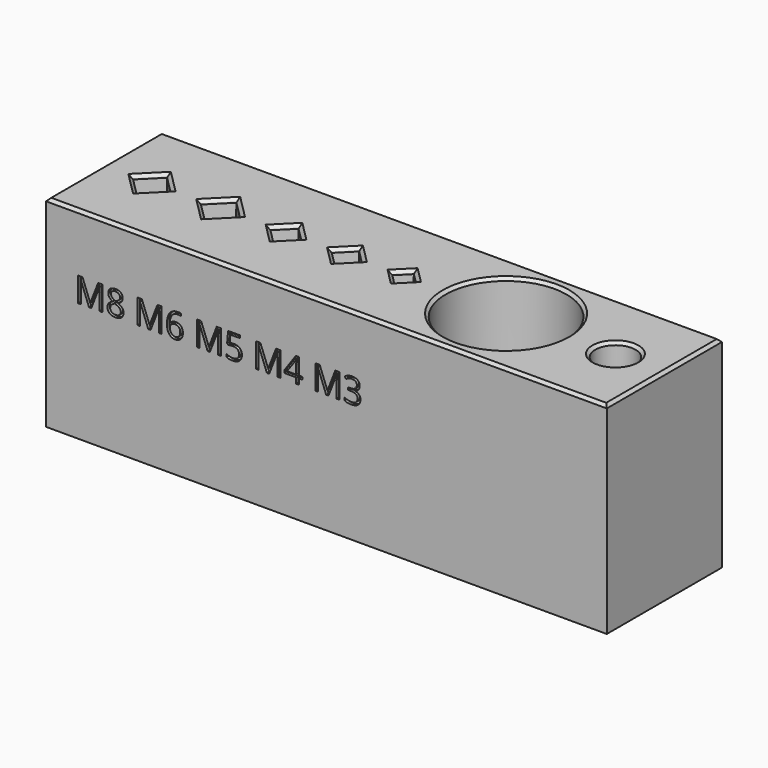
from build123d import *

# Parameters (mm, degrees)
F0_W          = 97.4156420974
F0_H          = 25
F0_R          = 10.5
F0_R_2        = 3.5
F1_DEPTH      = 13
F2_W          = 97.4156420974
F2_H          = 25
F2_R          = 10.5
F2_R_2        = 3.5
F3_DEPTH      = 20
F4_SIZE       = 0.5
F5_W          = 97.4156420974
F5_H          = 25
F6_DEPTH      = 2
F7_SIZE       = 3
F8_T4_DEPTH   = 49.6859183731
F8_T9_DEPTH   = 5
F8_T14_DEPTH  = 49.6859183731
F8_T19_DEPTH  = 49.6859183731
F8_T24_DEPTH  = 5
F8_T29_DEPTH  = 49.6859183731
F8_T34_DEPTH  = 49.6859183731
F8_T39_DEPTH  = 5
F8_T44_DEPTH  = 49.6859183731
F8_T49_DEPTH  = 49.6859183731
F8_T54_DEPTH  = 5
F8_T59_DEPTH  = 49.6859183731
F8_T64_DEPTH  = 48.6859183731
F8_T69_DEPTH  = 4
F8_T74_DEPTH  = 48.6859183731
F8_T79_DEPTH  = 48.6859183731
F8_T84_DEPTH  = 4
F8_T89_DEPTH  = 48.6859183731
F8_T94_DEPTH  = 48.6859183731
F8_T99_DEPTH  = 4
F8_T104_DEPTH = 48.6859183731
F8_T109_DEPTH = 48.6859183731
F8_T114_DEPTH = 4
F8_T119_DEPTH = 48.6859183731
F8_T124_DEPTH = 48.5859183731
F8_T129_DEPTH = 3.9
F8_T134_DEPTH = 48.5859183731
F8_T139_DEPTH = 48.5859183731
F8_T144_DEPTH = 3.9
F8_T149_DEPTH = 48.5859183731
F8_T154_DEPTH = 48.5859183731
F8_T159_DEPTH = 3.9
F8_T164_DEPTH = 48.5859183731
F8_T169_DEPTH = 48.5859183731
F8_T174_DEPTH = 3.9
F8_T179_DEPTH = 48.5859183731
F8_T184_DEPTH = 47.7859183731
F8_T189_DEPTH = 3.1
F8_T194_DEPTH = 47.7859183731
F8_T199_DEPTH = 47.7859183731
F8_T204_DEPTH = 3.1
F8_T209_DEPTH = 47.7859183731
F8_T214_DEPTH = 47.7859183731
F8_T219_DEPTH = 3.1
F8_T224_DEPTH = 47.7859183731
F8_T229_DEPTH = 47.7859183731
F8_T234_DEPTH = 3.1
F8_T239_DEPTH = 47.7859183731
F8_T244_DEPTH = 4.8
F8_T249_DEPTH = 4.8
F8_T254_DEPTH = 49.4859183731
F8_T259_DEPTH = 49.4859183731
F8_T264_DEPTH = 4.8
F8_T269_DEPTH = 49.4859183731
F8_T274_DEPTH = 49.4859183731
F8_T279_DEPTH = 4.8
F8_T284_DEPTH = 49.4859183731
F8_T289_DEPTH = 49.4859183731
F8_T294_DEPTH = 4.8
F8_T299_DEPTH = 4.8
F9_TEXT_SIZE  = 5.9394546838
F10_DEPTH     = 0.5


# Not quite as in the source:
# - a fillet or chamfer that OpenCascade refuses, or shapes differently, is made with other operations: its cross-section is extruded or revolved along the edge and cut away or added
# - Text() gives the source's letters only with a copy of the font that has no kerning and outlines rounded to 1/6400 em; it was checked with that copy


with BuildPart() as f1:
    # F0 (on Top) → F1 (new body)
    with BuildSketch(Plane.XY):
        with Locations((38.0792391653, 0)):
            Rectangle(F0_W, F0_H)
        Polygon((18.2307110279, 0), (21.0591381526, 2.8284271247), (23.8875652774, 0), (21.0591381526, -2.8284271247), align=None, mode=Mode.SUBTRACT)
        Polygon((-5.6285818834, 0), (-2.2344693337, 3.3941125497), (1.159643216, 0), (-2.2344693337, -3.3941125497), align=None, mode=Mode.SUBTRACT)
        Polygon((6.159643216, 0), (9.6951771219, 3.5355339059), (13.2307110279, 0), (9.6951771219, -3.5355339059), align=None, mode=Mode.SUBTRACT)
        Polygon((28.8875652774, 0), (31.645281724, 2.7577164466), (34.4029981706, 0), (31.645281724, -2.7577164466), align=None, mode=Mode.SUBTRACT)
        Polygon((39.4029981706, 0), (41.5950291923, 2.1920310217), (43.787060214, 0), (41.5950291923, -2.1920310217), align=None, mode=Mode.SUBTRACT)
        with Locations((59.287060214, 0)):
            Circle(F0_R, mode=Mode.SUBTRACT)
        with Locations((78.287060214, 0)):
            Circle(F0_R_2, mode=Mode.SUBTRACT)
    extrude(amount=F1_DEPTH)

    # F2 (on face) → F3 (join)
    with BuildSketch(Plane(origin=(0, 0, 0), x_dir=(1, 0, 0), z_dir=(0, 0, -1))):
        with Locations((38.0792391653, 0)):
            Rectangle(F2_W, F2_H)
        Polygon((1.159643216, 0), (-2.2344693337, -3.3941125497), (-5.6285818834, 0), (-2.2344693337, 3.3941125497), align=None, mode=Mode.SUBTRACT)
        Polygon((6.159643216, 0), (9.6951771219, 3.5355339059), (13.2307110279, 0), (9.6951771219, -3.5355339059), align=None, mode=Mode.SUBTRACT)
        Polygon((34.4029981706, 0), (31.645281724, -2.7577164466), (28.8875652774, 0), (31.645281724, 2.7577164466), align=None, mode=Mode.SUBTRACT)
        Polygon((41.5950291923, 2.1920310217), (43.787060214, 0), (41.5950291923, -2.1920310217), (39.4029981706, 0), align=None, mode=Mode.SUBTRACT)
        Polygon((23.8875652774, 0), (21.0591381526, -2.8284271247), (18.2307110279, 0), (21.0591381526, 2.8284271247), align=None, mode=Mode.SUBTRACT)
        with Locations((59.287060214, 0)):
            Circle(F2_R, mode=Mode.SUBTRACT)
        with Locations((78.287060214, 0)):
            Circle(F2_R_2, mode=Mode.SUBTRACT)
        Polygon((13.2307110279, 0), (9.6951771219, 3.5355339059), (6.159643216, 0), (9.6951771219, -3.5355339059), align=None)
        Polygon((-5.6285818834, 0), (-2.2344693337, -3.3941125497), (1.159643216, 0), (-2.2344693337, 3.3941125497), align=None)
        Polygon((18.2307110279, 0), (21.0591381526, -2.8284271247), (23.8875652774, 0), (21.0591381526, 2.8284271247), align=None)
        Polygon((28.8875652774, 0), (31.645281724, -2.7577164466), (34.4029981706, 0), (31.645281724, 2.7577164466), align=None)
        Polygon((41.5950291923, -2.1920310217), (43.787060214, 0), (41.5950291923, 2.1920310217), (39.4029981706, 0), align=None)
    extrude(amount=F3_DEPTH)

    # F4
    f4_edges = [f1.edges().sort_by_distance(p)[0] for p in [
        (38.079239, -12.5, 13),
        (86.78706, 0, 13),
        (38.079239, 12.5, 13),
        (-10.628582, 0, 13),
        (19.644925, 1.414214, 13),
        (22.473352, 1.414214, 13),
        (22.473352, -1.414214, 13),
        (19.644925, -1.414214, 13),
        (-3.931526, 1.697056, 13),
        (-0.537413, 1.697056, 13),
        (-0.537413, -1.697056, 13),
        (-3.931526, -1.697056, 13),
        (11.462944, -1.767767, 13),
        (7.92741, -1.767767, 13),
        (7.92741, 1.767767, 13),
        (11.462944, 1.767767, 13),
        (30.266424, 1.378858, 13),
        (33.02414, 1.378858, 13),
        (33.02414, -1.378858, 13),
        (30.266424, -1.378858, 13),
        (42.691045, 1.096016, 13),
        (42.691045, -1.096016, 13),
        (40.499014, -1.096016, 13),
        (40.499014, 1.096016, 13),
        (48.78706, 0, 13),
        (74.78706, 0, 13),
    ]]
    chamfer(f4_edges, length=F4_SIZE)

    # F5 (on face) → F6 (join)
    with BuildSketch(Plane(origin=(0, 0, -20), x_dir=(1, 0, 0), z_dir=(0, 0, -1))):
        with Locations((38.0792391653, 0)):
            Rectangle(F5_W, F5_H)
    extrude(amount=F6_DEPTH)

    # F7
    f7_edges = [f1.edges().sort_by_distance(p)[0] for p in [
        (48.78706, 0, -20),
    ]]
    chamfer(f7_edges, length=F7_SIZE)

    # F8: chamfer of 0.3 x 17.1869884892 on 21 edges, made by hand


with BuildPart() as f8_tool2:
    # F8_s3 → F8_t4 (new body)
    with BuildSketch(Plane(origin=(3.079821608, -3.079821608, 0), x_dir=(0, 0, 1), z_dir=(0.7071067812, -0.7071067812, 0))):
        Polygon((17.1869884892, -9.3555254877), (0, -9.0555254877), (0, -9.3555254877), align=None)
    extrude(amount=F8_T4_DEPTH)

    split(bisect_by=Plane(origin=(5.9593281864, -5.9593281864, 8.4277627439), x_dir=(-0.7071067812, -0.7071067812, 0), z_dir=(-0.5, 0.5, -0.7071067812)), keep=Keep.TOP)


with BuildPart() as f1_1:
    add(f1.part)

    # F8_t1: union F8_tool2
    add(f8_tool2.part)


with BuildPart() as f8_tool7:
    # F8_s8 → F8_t9 (new body)
    with BuildSketch(Plane(origin=(3.079821608, -3.079821608, 0), x_dir=(0, 0, 1), z_dir=(0.7071067812, -0.7071067812, 0))):
        Polygon((17.1869884892, -9.3555254877), (0, -9.0555254877), (0, -9.3555254877), align=None)
    extrude(amount=F8_T9_DEPTH)

    split(bisect_by=Plane(origin=(-1.1117396254, -1.1117396254, 1.5722372561), x_dir=(-0.7071067812, 0.7071067812, 0), z_dir=(0.5, 0.5, -0.7071067812)), keep=Keep.TOP)


with BuildPart() as f1_2:
    add(f1_1.part)

    # F8_t6: union F8_tool7
    add(f8_tool7.part)


with BuildPart() as f8_tool12:
    # F8_s13 → F8_t14 (new body)
    with BuildSketch(Plane(origin=(-28.5178942971, 28.5178942971, 0), x_dir=(0, 0, 1), z_dir=(0.7071067812, -0.7071067812, 0))):
        Polygon((17.1869884892, -9.3555254877), (0, -9.0555254877), (0, -9.3555254877), align=None)
    extrude(amount=F8_T14_DEPTH)

    split(bisect_by=Plane(origin=(-1.1117396254, 1.1117396254, 1.5722372561), x_dir=(0.7071067812, 0.7071067812, 0), z_dir=(0.5, -0.5, -0.7071067812)), keep=Keep.TOP)


with BuildPart() as f1_3:
    add(f1_2.part)

    # F8_t11: union F8_tool12
    add(f8_tool12.part)


with BuildPart() as f8_tool17:
    # F8_s18 → F8_t19 (new body)
    with BuildSketch(Plane(origin=(3.079821608, 3.079821608, 0), x_dir=(0, 0, 1), z_dir=(0.7071067812, 0.7071067812, 0))):
        Polygon((17.1869884892, 4.3555254877), (0, 4.6555254877), (0, 4.3555254877), align=None)
    extrude(amount=F8_T19_DEPTH)

    split(bisect_by=Plane(origin=(5.9593281864, 5.9593281864, 8.4277627439), x_dir=(0.7071067812, -0.7071067812, 0), z_dir=(-0.5, -0.5, -0.7071067812)), keep=Keep.TOP)


with BuildPart() as f1_4:
    add(f1_3.part)

    # F8_t16: union F8_tool17
    add(f8_tool17.part)


with BuildPart() as f8_tool22:
    # F8_s23 → F8_t24 (new body)
    with BuildSketch(Plane(origin=(3.079821608, 3.079821608, 0), x_dir=(0, 0, 1), z_dir=(0.7071067812, 0.7071067812, 0))):
        Polygon((17.1869884892, 4.3555254877), (0, 4.6555254877), (0, 4.3555254877), align=None)
    extrude(amount=F8_T24_DEPTH)

    split(bisect_by=Plane(origin=(5.9593281864, -5.9593281864, 8.4277627439), x_dir=(-0.7071067812, -0.7071067812, 0), z_dir=(-0.5, 0.5, -0.7071067812)), keep=Keep.TOP)


with BuildPart() as f1_5:
    add(f1_4.part)

    # F8_t21: union F8_tool22
    add(f8_tool22.part)


with BuildPart() as f8_tool27:
    # F8_s28 → F8_t29 (new body)
    with BuildSketch(Plane(origin=(-28.5178942971, -28.5178942971, 0), x_dir=(0, 0, 1), z_dir=(0.7071067812, 0.7071067812, 0))):
        Polygon((17.1869884892, 4.3555254877), (0, 4.6555254877), (0, 4.3555254877), align=None)
    extrude(amount=F8_T29_DEPTH)

    split(bisect_by=Plane(origin=(-1.1117396254, -1.1117396254, 1.5722372561), x_dir=(-0.7071067812, 0.7071067812, 0), z_dir=(0.5, 0.5, -0.7071067812)), keep=Keep.TOP)


with BuildPart() as f1_6:
    add(f1_5.part)

    # F8_t26: union F8_tool27
    add(f8_tool27.part)


with BuildPart() as f8_tool32:
    # F8_s33 → F8_t34 (new body)
    with BuildSketch(Plane(origin=(6.6153555139, -6.6153555139, 0), x_dir=(0, 0, 1), z_dir=(-0.7071067812, 0.7071067812, 0))):
        Polygon((17.1869884892, 4.3555254877), (0, 4.6555254877), (0, 4.3555254877), align=None)
    extrude(amount=F8_T34_DEPTH)

    split(bisect_by=Plane(origin=(-1.1117396254, 1.1117396254, 1.5722372561), x_dir=(0.7071067812, 0.7071067812, 0), z_dir=(0.5, -0.5, -0.7071067812)), keep=Keep.TOP)


with BuildPart() as f1_7:
    add(f1_6.part)

    # F8_t31: union F8_tool32
    add(f8_tool32.part)


with BuildPart() as f8_tool37:
    # F8_s38 → F8_t39 (new body)
    with BuildSketch(Plane(origin=(6.6153555139, -6.6153555139, 0), x_dir=(0, 0, 1), z_dir=(-0.7071067812, 0.7071067812, 0))):
        Polygon((17.1869884892, 4.3555254877), (0, 4.6555254877), (0, 4.3555254877), align=None)
    extrude(amount=F8_T39_DEPTH)

    split(bisect_by=Plane(origin=(5.9593281864, 5.9593281864, 8.4277627439), x_dir=(0.7071067812, -0.7071067812, 0), z_dir=(-0.5, -0.5, -0.7071067812)), keep=Keep.TOP)


with BuildPart() as f1_8:
    add(f1_7.part)

    # F8_t36: union F8_tool37
    add(f8_tool37.part)


with BuildPart() as f8_tool42:
    # F8_s43 → F8_t44 (new body)
    with BuildSketch(Plane(origin=(38.2130714191, -38.2130714191, 0), x_dir=(0, 0, 1), z_dir=(-0.7071067812, 0.7071067812, 0))):
        Polygon((17.1869884892, 4.3555254877), (0, 4.6555254877), (0, 4.3555254877), align=None)
    extrude(amount=F8_T44_DEPTH)

    split(bisect_by=Plane(origin=(5.9593281864, -5.9593281864, 8.4277627439), x_dir=(-0.7071067812, -0.7071067812, 0), z_dir=(-0.5, 0.5, -0.7071067812)), keep=Keep.TOP)


with BuildPart() as f1_9:
    add(f1_8.part)

    # F8_t41: union F8_tool42
    add(f8_tool42.part)


with BuildPart() as f8_tool47:
    # F8_s48 → F8_t49 (new body)
    with BuildSketch(Plane(origin=(6.6153555139, 6.6153555139, 0), x_dir=(0, 0, 1), z_dir=(-0.7071067812, -0.7071067812, 0))):
        Polygon((17.1869884892, -9.3555254877), (0, -9.0555254877), (0, -9.3555254877), align=None)
    extrude(amount=F8_T49_DEPTH)

    split(bisect_by=Plane(origin=(-1.1117396254, -1.1117396254, 1.5722372561), x_dir=(-0.7071067812, 0.7071067812, 0), z_dir=(0.5, 0.5, -0.7071067812)), keep=Keep.TOP)


with BuildPart() as f1_10:
    add(f1_9.part)

    # F8_t46: union F8_tool47
    add(f8_tool47.part)


with BuildPart() as f8_tool52:
    # F8_s53 → F8_t54 (new body)
    with BuildSketch(Plane(origin=(6.6153555139, 6.6153555139, 0), x_dir=(0, 0, 1), z_dir=(-0.7071067812, -0.7071067812, 0))):
        Polygon((17.1869884892, -9.3555254877), (0, -9.0555254877), (0, -9.3555254877), align=None)
    extrude(amount=F8_T54_DEPTH)

    split(bisect_by=Plane(origin=(-1.1117396254, 1.1117396254, 1.5722372561), x_dir=(0.7071067812, 0.7071067812, 0), z_dir=(0.5, -0.5, -0.7071067812)), keep=Keep.TOP)


with BuildPart() as f1_11:
    add(f1_10.part)

    # F8_t51: union F8_tool52
    add(f8_tool52.part)


with BuildPart() as f8_tool57:
    # F8_s58 → F8_t59 (new body)
    with BuildSketch(Plane(origin=(38.2130714191, 38.2130714191, 0), x_dir=(0, 0, 1), z_dir=(-0.7071067812, -0.7071067812, 0))):
        Polygon((17.1869884892, -9.3555254877), (0, -9.0555254877), (0, -9.3555254877), align=None)
    extrude(amount=F8_T59_DEPTH)

    split(bisect_by=Plane(origin=(5.9593281864, 5.9593281864, 8.4277627439), x_dir=(0.7071067812, -0.7071067812, 0), z_dir=(-0.5, -0.5, -0.7071067812)), keep=Keep.TOP)


with BuildPart() as f1_12:
    add(f1_11.part)

    # F8_t56: union F8_tool57
    add(f8_tool57.part)


with BuildPart() as f8_tool62:
    # F8_s63 → F8_t64 (new body)
    with BuildSketch(Plane(origin=(11.9437826387, -11.9437826387, 0), x_dir=(0, 0, 1), z_dir=(-0.7071067812, 0.7071067812, 0))):
        Polygon((17.1869884892, 12.8910593937), (0, 13.1910593937), (0, 12.8910593937), align=None)
    extrude(amount=F8_T64_DEPTH)

    split(bisect_by=Plane(origin=(1.5524739369, -1.5524739369, -2.1955296968), x_dir=(0.7071067812, 0.7071067812, 0), z_dir=(0.5, -0.5, -0.7071067812)), keep=Keep.TOP)


with BuildPart() as f1_13:
    add(f1_12.part)

    # F8_t61: union F8_tool62
    add(f8_tool62.part)


with BuildPart() as f8_tool67:
    # F8_s68 → F8_t69 (new body)
    with BuildSketch(Plane(origin=(11.9437826387, -11.9437826387, 0), x_dir=(0, 0, 1), z_dir=(-0.7071067812, 0.7071067812, 0))):
        Polygon((17.1869884892, 12.8910593937), (0, 13.1910593937), (0, 12.8910593937), align=None)
    extrude(amount=F8_T69_DEPTH)

    split(bisect_by=Plane(origin=(8.9770951394, 8.9770951394, 12.6955296968), x_dir=(0.7071067812, -0.7071067812, 0), z_dir=(-0.5, -0.5, -0.7071067812)), keep=Keep.TOP)


with BuildPart() as f1_14:
    add(f1_13.part)

    # F8_t66: union F8_tool67
    add(f8_tool67.part)


with BuildPart() as f8_tool72:
    # F8_s73 → F8_t74 (new body)
    with BuildSketch(Plane(origin=(43.5414985438, -43.5414985438, 0), x_dir=(0, 0, 1), z_dir=(-0.7071067812, 0.7071067812, 0))):
        Polygon((17.1869884892, 12.8910593937), (0, 13.1910593937), (0, 12.8910593937), align=None)
    extrude(amount=F8_T74_DEPTH)

    split(bisect_by=Plane(origin=(8.9770951394, -8.9770951394, 12.6955296968), x_dir=(-0.7071067812, -0.7071067812, 0), z_dir=(-0.5, 0.5, -0.7071067812)), keep=Keep.TOP)


with BuildPart() as f1_15:
    add(f1_14.part)

    # F8_t71: union F8_tool72
    add(f8_tool72.part)


with BuildPart() as f8_tool77:
    # F8_s78 → F8_t79 (new body)
    with BuildSketch(Plane(origin=(11.9437826387, 11.9437826387, 0), x_dir=(0, 0, 1), z_dir=(-0.7071067812, -0.7071067812, 0))):
        Polygon((17.1869884892, -16.8910593937), (0, -16.5910593937), (0, -16.8910593937), align=None)
    extrude(amount=F8_T79_DEPTH)

    split(bisect_by=Plane(origin=(1.5524739369, 1.5524739369, -2.1955296968), x_dir=(-0.7071067812, 0.7071067812, 0), z_dir=(0.5, 0.5, -0.7071067812)), keep=Keep.TOP)


with BuildPart() as f1_16:
    add(f1_15.part)

    # F8_t76: union F8_tool77
    add(f8_tool77.part)


with BuildPart() as f8_tool82:
    # F8_s83 → F8_t84 (new body)
    with BuildSketch(Plane(origin=(11.9437826387, 11.9437826387, 0), x_dir=(0, 0, 1), z_dir=(-0.7071067812, -0.7071067812, 0))):
        Polygon((17.1869884892, -16.8910593937), (0, -16.5910593937), (0, -16.8910593937), align=None)
    extrude(amount=F8_T84_DEPTH)

    split(bisect_by=Plane(origin=(1.5524739369, -1.5524739369, -2.1955296968), x_dir=(0.7071067812, 0.7071067812, 0), z_dir=(0.5, -0.5, -0.7071067812)), keep=Keep.TOP)


with BuildPart() as f1_17:
    add(f1_16.part)

    # F8_t81: union F8_tool82
    add(f8_tool82.part)


with BuildPart() as f8_tool87:
    # F8_s88 → F8_t89 (new body)
    with BuildSketch(Plane(origin=(43.5414985438, 43.5414985438, 0), x_dir=(0, 0, 1), z_dir=(-0.7071067812, -0.7071067812, 0))):
        Polygon((17.1869884892, -16.8910593937), (0, -16.5910593937), (0, -16.8910593937), align=None)
    extrude(amount=F8_T89_DEPTH)

    split(bisect_by=Plane(origin=(8.9770951394, 8.9770951394, 12.6955296968), x_dir=(0.7071067812, -0.7071067812, 0), z_dir=(-0.5, -0.5, -0.7071067812)), keep=Keep.TOP)


with BuildPart() as f1_18:
    add(f1_17.part)

    # F8_t86: union F8_tool87
    add(f8_tool87.part)


with BuildPart() as f8_tool92:
    # F8_s93 → F8_t94 (new body)
    with BuildSketch(Plane(origin=(9.1153555139, -9.1153555139, 0), x_dir=(0, 0, 1), z_dir=(0.7071067812, -0.7071067812, 0))):
        Polygon((17.1869884892, -16.8910593937), (0, -16.5910593937), (0, -16.8910593937), align=None)
    extrude(amount=F8_T94_DEPTH)

    split(bisect_by=Plane(origin=(8.9770951394, -8.9770951394, 12.6955296968), x_dir=(-0.7071067812, -0.7071067812, 0), z_dir=(-0.5, 0.5, -0.7071067812)), keep=Keep.TOP)


with BuildPart() as f1_19:
    add(f1_18.part)

    # F8_t91: union F8_tool92
    add(f8_tool92.part)


with BuildPart() as f8_tool97:
    # F8_s98 → F8_t99 (new body)
    with BuildSketch(Plane(origin=(9.1153555139, -9.1153555139, 0), x_dir=(0, 0, 1), z_dir=(0.7071067812, -0.7071067812, 0))):
        Polygon((17.1869884892, -16.8910593937), (0, -16.5910593937), (0, -16.8910593937), align=None)
    extrude(amount=F8_T99_DEPTH)

    split(bisect_by=Plane(origin=(1.5524739369, 1.5524739369, -2.1955296968), x_dir=(-0.7071067812, 0.7071067812, 0), z_dir=(0.5, 0.5, -0.7071067812)), keep=Keep.TOP)


with BuildPart() as f1_20:
    add(f1_19.part)

    # F8_t96: union F8_tool97
    add(f8_tool97.part)


with BuildPart() as f8_tool102:
    # F8_s103 → F8_t104 (new body)
    with BuildSketch(Plane(origin=(-22.4823603912, 22.4823603912, 0), x_dir=(0, 0, 1), z_dir=(0.7071067812, -0.7071067812, 0))):
        Polygon((17.1869884892, -16.8910593937), (0, -16.5910593937), (0, -16.8910593937), align=None)
    extrude(amount=F8_T104_DEPTH)

    split(bisect_by=Plane(origin=(1.5524739369, -1.5524739369, -2.1955296968), x_dir=(0.7071067812, 0.7071067812, 0), z_dir=(0.5, -0.5, -0.7071067812)), keep=Keep.TOP)


with BuildPart() as f1_21:
    add(f1_20.part)

    # F8_t101: union F8_tool102
    add(f8_tool102.part)


with BuildPart() as f8_tool107:
    # F8_s108 → F8_t109 (new body)
    with BuildSketch(Plane(origin=(9.1153555139, 9.1153555139, 0), x_dir=(0, 0, 1), z_dir=(0.7071067812, 0.7071067812, 0))):
        Polygon((17.1869884892, 12.8910593937), (0, 13.1910593937), (0, 12.8910593937), align=None)
    extrude(amount=F8_T109_DEPTH)

    split(bisect_by=Plane(origin=(8.9770951394, 8.9770951394, 12.6955296968), x_dir=(0.7071067812, -0.7071067812, 0), z_dir=(-0.5, -0.5, -0.7071067812)), keep=Keep.TOP)


with BuildPart() as f1_22:
    add(f1_21.part)

    # F8_t106: union F8_tool107
    add(f8_tool107.part)


with BuildPart() as f8_tool112:
    # F8_s113 → F8_t114 (new body)
    with BuildSketch(Plane(origin=(9.1153555139, 9.1153555139, 0), x_dir=(0, 0, 1), z_dir=(0.7071067812, 0.7071067812, 0))):
        Polygon((17.1869884892, 12.8910593937), (0, 13.1910593937), (0, 12.8910593937), align=None)
    extrude(amount=F8_T114_DEPTH)

    split(bisect_by=Plane(origin=(8.9770951394, -8.9770951394, 12.6955296968), x_dir=(-0.7071067812, -0.7071067812, 0), z_dir=(-0.5, 0.5, -0.7071067812)), keep=Keep.TOP)


with BuildPart() as f1_23:
    add(f1_22.part)

    # F8_t111: union F8_tool112
    add(f8_tool112.part)


with BuildPart() as f8_tool117:
    # F8_s118 → F8_t119 (new body)
    with BuildSketch(Plane(origin=(-22.4823603912, -22.4823603912, 0), x_dir=(0, 0, 1), z_dir=(0.7071067812, 0.7071067812, 0))):
        Polygon((17.1869884892, 12.8910593937), (0, 13.1910593937), (0, 12.8910593937), align=None)
    extrude(amount=F8_T119_DEPTH)

    split(bisect_by=Plane(origin=(1.5524739369, 1.5524739369, -2.1955296968), x_dir=(-0.7071067812, 0.7071067812, 0), z_dir=(0.5, 0.5, -0.7071067812)), keep=Keep.TOP)


with BuildPart() as f1_24:
    add(f1_23.part)

    # F8_t116: union F8_tool117
    add(f8_tool117.part)


with BuildPart() as f8_tool122:
    # F8_s123 → F8_t124 (new body)
    with BuildSketch(Plane(origin=(17.2014990853, -17.2014990853, 0), x_dir=(0, 0, 1), z_dir=(-0.7071067812, 0.7071067812, 0))):
        Polygon((17.1869884892, 20.4265932996), (0, 20.7265932996), (0, 20.4265932996), align=None)
    extrude(amount=F8_T124_DEPTH)

    split(bisect_by=Plane(origin=(4.1813321602, -4.1813321602, -5.9132966498), x_dir=(0.7071067812, 0.7071067812, 0), z_dir=(0.5, -0.5, -0.7071067812)), keep=Keep.TOP)


with BuildPart() as f1_25:
    add(f1_24.part)

    # F8_t121: union F8_tool122
    add(f8_tool122.part)


with BuildPart() as f8_tool127:
    # F8_s128 → F8_t129 (new body)
    with BuildSketch(Plane(origin=(17.2014990853, -17.2014990853, 0), x_dir=(0, 0, 1), z_dir=(-0.7071067812, 0.7071067812, 0))):
        Polygon((17.1869884892, 20.4265932996), (0, 20.7265932996), (0, 20.4265932996), align=None)
    extrude(amount=F8_T129_DEPTH)

    split(bisect_by=Plane(origin=(11.6413087018, 11.6413087018, 16.4632966498), x_dir=(0.7071067812, -0.7071067812, 0), z_dir=(-0.5, -0.5, -0.7071067812)), keep=Keep.TOP)


with BuildPart() as f1_26:
    add(f1_25.part)

    # F8_t126: union F8_tool127
    add(f8_tool127.part)


with BuildPart() as f8_tool132:
    # F8_s133 → F8_t134 (new body)
    with BuildSketch(Plane(origin=(48.7992149904, -48.7992149904, 0), x_dir=(0, 0, 1), z_dir=(-0.7071067812, 0.7071067812, 0))):
        Polygon((17.1869884892, 20.4265932996), (0, 20.7265932996), (0, 20.4265932996), align=None)
    extrude(amount=F8_T134_DEPTH)

    split(bisect_by=Plane(origin=(11.6413087018, -11.6413087018, 16.4632966498), x_dir=(-0.7071067812, -0.7071067812, 0), z_dir=(-0.5, 0.5, -0.7071067812)), keep=Keep.TOP)


with BuildPart() as f1_27:
    add(f1_26.part)

    # F8_t131: union F8_tool132
    add(f8_tool132.part)


with BuildPart() as f8_tool137:
    # F8_s138 → F8_t139 (new body)
    with BuildSketch(Plane(origin=(17.2014990853, 17.2014990853, 0), x_dir=(0, 0, 1), z_dir=(-0.7071067812, -0.7071067812, 0))):
        Polygon((17.1869884892, -24.3265932996), (0, -24.0265932996), (0, -24.3265932996), align=None)
    extrude(amount=F8_T139_DEPTH)

    split(bisect_by=Plane(origin=(4.1813321602, 4.1813321602, -5.9132966498), x_dir=(-0.7071067812, 0.7071067812, 0), z_dir=(0.5, 0.5, -0.7071067812)), keep=Keep.TOP)


with BuildPart() as f1_28:
    add(f1_27.part)

    # F8_t136: union F8_tool137
    add(f8_tool137.part)


with BuildPart() as f8_tool142:
    # F8_s143 → F8_t144 (new body)
    with BuildSketch(Plane(origin=(17.2014990853, 17.2014990853, 0), x_dir=(0, 0, 1), z_dir=(-0.7071067812, -0.7071067812, 0))):
        Polygon((17.1869884892, -24.3265932996), (0, -24.0265932996), (0, -24.3265932996), align=None)
    extrude(amount=F8_T144_DEPTH)

    split(bisect_by=Plane(origin=(4.1813321602, -4.1813321602, -5.9132966498), x_dir=(0.7071067812, 0.7071067812, 0), z_dir=(0.5, -0.5, -0.7071067812)), keep=Keep.TOP)


with BuildPart() as f1_29:
    add(f1_28.part)

    # F8_t141: union F8_tool142
    add(f8_tool142.part)


with BuildPart() as f8_tool147:
    # F8_s148 → F8_t149 (new body)
    with BuildSketch(Plane(origin=(48.7992149904, 48.7992149904, 0), x_dir=(0, 0, 1), z_dir=(-0.7071067812, -0.7071067812, 0))):
        Polygon((17.1869884892, -24.3265932996), (0, -24.0265932996), (0, -24.3265932996), align=None)
    extrude(amount=F8_T149_DEPTH)

    split(bisect_by=Plane(origin=(11.6413087018, 11.6413087018, 16.4632966498), x_dir=(0.7071067812, -0.7071067812, 0), z_dir=(-0.5, -0.5, -0.7071067812)), keep=Keep.TOP)


with BuildPart() as f1_30:
    add(f1_29.part)

    # F8_t146: union F8_tool147
    add(f8_tool147.part)


with BuildPart() as f8_tool152:
    # F8_s153 → F8_t154 (new body)
    with BuildSketch(Plane(origin=(14.4437826387, -14.4437826387, 0), x_dir=(0, 0, 1), z_dir=(0.7071067812, -0.7071067812, 0))):
        Polygon((17.1869884892, -24.3265932996), (0, -24.0265932996), (0, -24.3265932996), align=None)
    extrude(amount=F8_T154_DEPTH)

    split(bisect_by=Plane(origin=(11.6413087018, -11.6413087018, 16.4632966498), x_dir=(-0.7071067812, -0.7071067812, 0), z_dir=(-0.5, 0.5, -0.7071067812)), keep=Keep.TOP)


with BuildPart() as f1_31:
    add(f1_30.part)

    # F8_t151: union F8_tool152
    add(f8_tool152.part)


with BuildPart() as f8_tool157:
    # F8_s158 → F8_t159 (new body)
    with BuildSketch(Plane(origin=(14.4437826387, -14.4437826387, 0), x_dir=(0, 0, 1), z_dir=(0.7071067812, -0.7071067812, 0))):
        Polygon((17.1869884892, -24.3265932996), (0, -24.0265932996), (0, -24.3265932996), align=None)
    extrude(amount=F8_T159_DEPTH)

    split(bisect_by=Plane(origin=(4.1813321602, 4.1813321602, -5.9132966498), x_dir=(-0.7071067812, 0.7071067812, 0), z_dir=(0.5, 0.5, -0.7071067812)), keep=Keep.TOP)


with BuildPart() as f1_32:
    add(f1_31.part)

    # F8_t156: union F8_tool157
    add(f8_tool157.part)


with BuildPart() as f8_tool162:
    # F8_s163 → F8_t164 (new body)
    with BuildSketch(Plane(origin=(-17.1539332665, 17.1539332665, 0), x_dir=(0, 0, 1), z_dir=(0.7071067812, -0.7071067812, 0))):
        Polygon((17.1869884892, -24.3265932996), (0, -24.0265932996), (0, -24.3265932996), align=None)
    extrude(amount=F8_T164_DEPTH)

    split(bisect_by=Plane(origin=(4.1813321602, -4.1813321602, -5.9132966498), x_dir=(0.7071067812, 0.7071067812, 0), z_dir=(0.5, -0.5, -0.7071067812)), keep=Keep.TOP)


with BuildPart() as f1_33:
    add(f1_32.part)

    # F8_t161: union F8_tool162
    add(f8_tool162.part)


with BuildPart() as f8_tool167:
    # F8_s168 → F8_t169 (new body)
    with BuildSketch(Plane(origin=(14.4437826387, 14.4437826387, 0), x_dir=(0, 0, 1), z_dir=(0.7071067812, 0.7071067812, 0))):
        Polygon((17.1869884892, 20.4265932996), (0, 20.7265932996), (0, 20.4265932996), align=None)
    extrude(amount=F8_T169_DEPTH)

    split(bisect_by=Plane(origin=(11.6413087018, 11.6413087018, 16.4632966498), x_dir=(0.7071067812, -0.7071067812, 0), z_dir=(-0.5, -0.5, -0.7071067812)), keep=Keep.TOP)


with BuildPart() as f1_34:
    add(f1_33.part)

    # F8_t166: union F8_tool167
    add(f8_tool167.part)


with BuildPart() as f8_tool172:
    # F8_s173 → F8_t174 (new body)
    with BuildSketch(Plane(origin=(14.4437826387, 14.4437826387, 0), x_dir=(0, 0, 1), z_dir=(0.7071067812, 0.7071067812, 0))):
        Polygon((17.1869884892, 20.4265932996), (0, 20.7265932996), (0, 20.4265932996), align=None)
    extrude(amount=F8_T174_DEPTH)

    split(bisect_by=Plane(origin=(11.6413087018, -11.6413087018, 16.4632966498), x_dir=(-0.7071067812, -0.7071067812, 0), z_dir=(-0.5, 0.5, -0.7071067812)), keep=Keep.TOP)


with BuildPart() as f1_35:
    add(f1_34.part)

    # F8_t171: union F8_tool172
    add(f8_tool172.part)


with BuildPart() as f8_tool177:
    # F8_s178 → F8_t179 (new body)
    with BuildSketch(Plane(origin=(-17.1539332665, -17.1539332665, 0), x_dir=(0, 0, 1), z_dir=(0.7071067812, 0.7071067812, 0))):
        Polygon((17.1869884892, 20.4265932996), (0, 20.7265932996), (0, 20.4265932996), align=None)
    extrude(amount=F8_T179_DEPTH)

    split(bisect_by=Plane(origin=(4.1813321602, 4.1813321602, -5.9132966498), x_dir=(-0.7071067812, 0.7071067812, 0), z_dir=(0.5, 0.5, -0.7071067812)), keep=Keep.TOP)


with BuildPart() as f1_36:
    add(f1_35.part)

    # F8_t176: union F8_tool177
    add(f8_tool177.part)


with BuildPart() as f8_tool182:
    # F8_s183 → F8_t184 (new body)
    with BuildSketch(Plane(origin=(19.7014990853, 19.7014990853, 0), x_dir=(0, 0, 1), z_dir=(0.7071067812, 0.7071067812, 0))):
        Polygon((17.1869884892, 27.8621272055), (0, 28.1621272055), (0, 27.8621272055), align=None)
    extrude(amount=F8_T184_DEPTH)

    split(bisect_by=Plane(origin=(14.2701669251, 14.2701669251, 20.1810636028), x_dir=(0.7071067812, -0.7071067812, 0), z_dir=(-0.5, -0.5, -0.7071067812)), keep=Keep.TOP)


with BuildPart() as f1_37:
    add(f1_36.part)

    # F8_t181: union F8_tool182
    add(f8_tool182.part)


with BuildPart() as f8_tool187:
    # F8_s188 → F8_t189 (new body)
    with BuildSketch(Plane(origin=(19.7014990853, 19.7014990853, 0), x_dir=(0, 0, 1), z_dir=(0.7071067812, 0.7071067812, 0))):
        Polygon((17.1869884892, 27.8621272055), (0, 28.1621272055), (0, 27.8621272055), align=None)
    extrude(amount=F8_T189_DEPTH)

    split(bisect_by=Plane(origin=(14.2701669251, -14.2701669251, 20.1810636028), x_dir=(-0.7071067812, -0.7071067812, 0), z_dir=(-0.5, 0.5, -0.7071067812)), keep=Keep.TOP)


with BuildPart() as f1_38:
    add(f1_37.part)

    # F8_t186: union F8_tool187
    add(f8_tool187.part)


with BuildPart() as f8_tool192:
    # F8_s193 → F8_t194 (new body)
    with BuildSketch(Plane(origin=(-11.8962168198, -11.8962168198, 0), x_dir=(0, 0, 1), z_dir=(0.7071067812, 0.7071067812, 0))):
        Polygon((17.1869884892, 27.8621272055), (0, 28.1621272055), (0, 27.8621272055), align=None)
    extrude(amount=F8_T194_DEPTH)

    split(bisect_by=Plane(origin=(6.5273476711, 6.5273476711, -9.2310636028), x_dir=(-0.7071067812, 0.7071067812, 0), z_dir=(0.5, 0.5, -0.7071067812)), keep=Keep.TOP)


with BuildPart() as f1_39:
    add(f1_38.part)

    # F8_t191: union F8_tool192
    add(f8_tool192.part)


with BuildPart() as f8_tool197:
    # F8_s198 → F8_t199 (new body)
    with BuildSketch(Plane(origin=(21.893530107, -21.893530107, 0), x_dir=(0, 0, 1), z_dir=(-0.7071067812, 0.7071067812, 0))):
        Polygon((17.1869884892, 27.8621272055), (0, 28.1621272055), (0, 27.8621272055), align=None)
    extrude(amount=F8_T199_DEPTH)

    split(bisect_by=Plane(origin=(6.5273476711, -6.5273476711, -9.2310636028), x_dir=(0.7071067812, 0.7071067812, 0), z_dir=(0.5, -0.5, -0.7071067812)), keep=Keep.TOP)


with BuildPart() as f1_40:
    add(f1_39.part)

    # F8_t196: union F8_tool197
    add(f8_tool197.part)


with BuildPart() as f8_tool202:
    # F8_s203 → F8_t204 (new body)
    with BuildSketch(Plane(origin=(21.893530107, -21.893530107, 0), x_dir=(0, 0, 1), z_dir=(-0.7071067812, 0.7071067812, 0))):
        Polygon((17.1869884892, 27.8621272055), (0, 28.1621272055), (0, 27.8621272055), align=None)
    extrude(amount=F8_T204_DEPTH)

    split(bisect_by=Plane(origin=(14.2701669251, 14.2701669251, 20.1810636028), x_dir=(0.7071067812, -0.7071067812, 0), z_dir=(-0.5, -0.5, -0.7071067812)), keep=Keep.TOP)


with BuildPart() as f1_41:
    add(f1_40.part)

    # F8_t201: union F8_tool202
    add(f8_tool202.part)


with BuildPart() as f8_tool207:
    # F8_s208 → F8_t209 (new body)
    with BuildSketch(Plane(origin=(53.4912460121, -53.4912460121, 0), x_dir=(0, 0, 1), z_dir=(-0.7071067812, 0.7071067812, 0))):
        Polygon((17.1869884892, 27.8621272055), (0, 28.1621272055), (0, 27.8621272055), align=None)
    extrude(amount=F8_T209_DEPTH)

    split(bisect_by=Plane(origin=(14.2701669251, -14.2701669251, 20.1810636028), x_dir=(-0.7071067812, -0.7071067812, 0), z_dir=(-0.5, 0.5, -0.7071067812)), keep=Keep.TOP)


with BuildPart() as f1_42:
    add(f1_41.part)

    # F8_t206: union F8_tool207
    add(f8_tool207.part)


with BuildPart() as f8_tool212:
    # F8_s213 → F8_t214 (new body)
    with BuildSketch(Plane(origin=(21.893530107, 21.893530107, 0), x_dir=(0, 0, 1), z_dir=(-0.7071067812, -0.7071067812, 0))):
        Polygon((17.1869884892, -30.9621272055), (0, -30.6621272055), (0, -30.9621272055), align=None)
    extrude(amount=F8_T214_DEPTH)

    split(bisect_by=Plane(origin=(6.5273476711, 6.5273476711, -9.2310636028), x_dir=(-0.7071067812, 0.7071067812, 0), z_dir=(0.5, 0.5, -0.7071067812)), keep=Keep.TOP)


with BuildPart() as f1_43:
    add(f1_42.part)

    # F8_t211: union F8_tool212
    add(f8_tool212.part)


with BuildPart() as f8_tool217:
    # F8_s218 → F8_t219 (new body)
    with BuildSketch(Plane(origin=(21.893530107, 21.893530107, 0), x_dir=(0, 0, 1), z_dir=(-0.7071067812, -0.7071067812, 0))):
        Polygon((17.1869884892, -30.9621272055), (0, -30.6621272055), (0, -30.9621272055), align=None)
    extrude(amount=F8_T219_DEPTH)

    split(bisect_by=Plane(origin=(6.5273476711, -6.5273476711, -9.2310636028), x_dir=(0.7071067812, 0.7071067812, 0), z_dir=(0.5, -0.5, -0.7071067812)), keep=Keep.TOP)


with BuildPart() as f1_44:
    add(f1_43.part)

    # F8_t216: union F8_tool217
    add(f8_tool217.part)


with BuildPart() as f8_tool222:
    # F8_s223 → F8_t224 (new body)
    with BuildSketch(Plane(origin=(53.4912460121, 53.4912460121, 0), x_dir=(0, 0, 1), z_dir=(-0.7071067812, -0.7071067812, 0))):
        Polygon((17.1869884892, -30.9621272055), (0, -30.6621272055), (0, -30.9621272055), align=None)
    extrude(amount=F8_T224_DEPTH)

    split(bisect_by=Plane(origin=(14.2701669251, 14.2701669251, 20.1810636028), x_dir=(0.7071067812, -0.7071067812, 0), z_dir=(-0.5, -0.5, -0.7071067812)), keep=Keep.TOP)


with BuildPart() as f1_45:
    add(f1_44.part)

    # F8_t221: union F8_tool222
    add(f8_tool222.part)


with BuildPart() as f8_tool227:
    # F8_s228 → F8_t229 (new body)
    with BuildSketch(Plane(origin=(19.7014990853, -19.7014990853, 0), x_dir=(0, 0, 1), z_dir=(0.7071067812, -0.7071067812, 0))):
        Polygon((17.1869884892, -30.9621272055), (0, -30.6621272055), (0, -30.9621272055), align=None)
    extrude(amount=F8_T229_DEPTH)

    split(bisect_by=Plane(origin=(14.2701669251, -14.2701669251, 20.1810636028), x_dir=(-0.7071067812, -0.7071067812, 0), z_dir=(-0.5, 0.5, -0.7071067812)), keep=Keep.TOP)


with BuildPart() as f1_46:
    add(f1_45.part)

    # F8_t226: union F8_tool227
    add(f8_tool227.part)


with BuildPart() as f8_tool232:
    # F8_s233 → F8_t234 (new body)
    with BuildSketch(Plane(origin=(19.7014990853, -19.7014990853, 0), x_dir=(0, 0, 1), z_dir=(0.7071067812, -0.7071067812, 0))):
        Polygon((17.1869884892, -30.9621272055), (0, -30.6621272055), (0, -30.9621272055), align=None)
    extrude(amount=F8_T234_DEPTH)

    split(bisect_by=Plane(origin=(6.5273476711, 6.5273476711, -9.2310636028), x_dir=(-0.7071067812, 0.7071067812, 0), z_dir=(0.5, 0.5, -0.7071067812)), keep=Keep.TOP)


with BuildPart() as f1_47:
    add(f1_46.part)

    # F8_t231: union F8_tool232
    add(f8_tool232.part)


with BuildPart() as f8_tool237:
    # F8_s238 → F8_t239 (new body)
    with BuildSketch(Plane(origin=(-11.8962168198, 11.8962168198, 0), x_dir=(0, 0, 1), z_dir=(0.7071067812, -0.7071067812, 0))):
        Polygon((17.1869884892, -30.9621272055), (0, -30.6621272055), (0, -30.9621272055), align=None)
    extrude(amount=F8_T239_DEPTH)

    split(bisect_by=Plane(origin=(6.5273476711, -6.5273476711, -9.2310636028), x_dir=(0.7071067812, 0.7071067812, 0), z_dir=(0.5, -0.5, -0.7071067812)), keep=Keep.TOP)


with BuildPart() as f1_48:
    add(f1_47.part)

    # F8_t236: union F8_tool237
    add(f8_tool237.part)


with BuildPart() as f8_tool242:
    # F8_s243 → F8_t244 (new body)
    with BuildSketch(Plane(origin=(0.579821608, -0.579821608, 0), x_dir=(0, 0, 1), z_dir=(-0.7071067812, 0.7071067812, 0))):
        Polygon((17.1869884892, -3.9800084182), (0, -3.6800084182), (0, -3.9800084182), align=None)
    extrude(amount=F8_T244_DEPTH)

    split(bisect_by=Plane(origin=(-4.1295065784, 4.1295065784, 5.8400042091), x_dir=(0.7071067812, 0.7071067812, 0), z_dir=(0.5, -0.5, -0.7071067812)), keep=Keep.TOP)


with BuildPart() as f1_49:
    add(f1_48.part)

    # F8_t241: union F8_tool242
    add(f8_tool242.part)


with BuildPart() as f8_tool247:
    # F8_s248 → F8_t249 (new body)
    with BuildSketch(Plane(origin=(0.579821608, -0.579821608, 0), x_dir=(0, 0, 1), z_dir=(-0.7071067812, 0.7071067812, 0))):
        Polygon((17.1869884892, -3.9800084182), (0, -3.6800084182), (0, -3.9800084182), align=None)
    extrude(amount=F8_T249_DEPTH)

    split(bisect_by=Plane(origin=(3.0122719116, 3.0122719116, 4.2599957909), x_dir=(0.7071067812, -0.7071067812, 0), z_dir=(-0.5, -0.5, -0.7071067812)), keep=Keep.TOP)


with BuildPart() as f1_50:
    add(f1_49.part)

    # F8_t246: union F8_tool247
    add(f8_tool247.part)


with BuildPart() as f8_tool252:
    # F8_s253 → F8_t254 (new body)
    with BuildSketch(Plane(origin=(32.1775375131, -32.1775375131, 0), x_dir=(0, 0, 1), z_dir=(-0.7071067812, 0.7071067812, 0))):
        Polygon((17.1869884892, -3.9800084182), (0, -3.6800084182), (0, -3.9800084182), align=None)
    extrude(amount=F8_T254_DEPTH)

    split(bisect_by=Plane(origin=(3.0122719116, -3.0122719116, 4.2599957909), x_dir=(-0.7071067812, -0.7071067812, 0), z_dir=(-0.5, 0.5, -0.7071067812)), keep=Keep.TOP)


with BuildPart() as f1_51:
    add(f1_50.part)

    # F8_t251: union F8_tool252
    add(f8_tool252.part)


with BuildPart() as f8_tool257:
    # F8_s258 → F8_t259 (new body)
    with BuildSketch(Plane(origin=(0.579821608, 0.579821608, 0), x_dir=(0, 0, 1), z_dir=(-0.7071067812, -0.7071067812, 0))):
        Polygon((17.1869884892, -0.8199915818), (0, -0.5199915818), (0, -0.8199915818), align=None)
    extrude(amount=F8_T259_DEPTH)

    split(bisect_by=Plane(origin=(-4.1295065784, -4.1295065784, 5.8400042091), x_dir=(-0.7071067812, 0.7071067812, 0), z_dir=(0.5, 0.5, -0.7071067812)), keep=Keep.TOP)


with BuildPart() as f1_52:
    add(f1_51.part)

    # F8_t256: union F8_tool257
    add(f8_tool257.part)


with BuildPart() as f8_tool262:
    # F8_s263 → F8_t264 (new body)
    with BuildSketch(Plane(origin=(0.579821608, 0.579821608, 0), x_dir=(0, 0, 1), z_dir=(-0.7071067812, -0.7071067812, 0))):
        Polygon((17.1869884892, -0.8199915818), (0, -0.5199915818), (0, -0.8199915818), align=None)
    extrude(amount=F8_T264_DEPTH)

    split(bisect_by=Plane(origin=(-4.1295065784, 4.1295065784, 5.8400042091), x_dir=(0.7071067812, 0.7071067812, 0), z_dir=(0.5, -0.5, -0.7071067812)), keep=Keep.TOP)


with BuildPart() as f1_53:
    add(f1_52.part)

    # F8_t261: union F8_tool262
    add(f8_tool262.part)


with BuildPart() as f8_tool267:
    # F8_s268 → F8_t269 (new body)
    with BuildSketch(Plane(origin=(32.1775375131, 32.1775375131, 0), x_dir=(0, 0, 1), z_dir=(-0.7071067812, -0.7071067812, 0))):
        Polygon((17.1869884892, -0.8199915818), (0, -0.5199915818), (0, -0.8199915818), align=None)
    extrude(amount=F8_T269_DEPTH)

    split(bisect_by=Plane(origin=(3.0122719116, 3.0122719116, 4.2599957909), x_dir=(0.7071067812, -0.7071067812, 0), z_dir=(-0.5, -0.5, -0.7071067812)), keep=Keep.TOP)


with BuildPart() as f1_54:
    add(f1_53.part)

    # F8_t266: union F8_tool267
    add(f8_tool267.part)


with BuildPart() as f8_tool272:
    # F8_s273 → F8_t274 (new body)
    with BuildSketch(Plane(origin=(-2.8142909417, 2.8142909417, 0), x_dir=(0, 0, 1), z_dir=(0.7071067812, -0.7071067812, 0))):
        Polygon((17.1869884892, -0.8199915818), (0, -0.5199915818), (0, -0.8199915818), align=None)
    extrude(amount=F8_T274_DEPTH)

    split(bisect_by=Plane(origin=(3.0122719116, -3.0122719116, 4.2599957909), x_dir=(-0.7071067812, -0.7071067812, 0), z_dir=(-0.5, 0.5, -0.7071067812)), keep=Keep.TOP)


with BuildPart() as f1_55:
    add(f1_54.part)

    # F8_t271: union F8_tool272
    add(f8_tool272.part)


with BuildPart() as f8_tool277:
    # F8_s278 → F8_t279 (new body)
    with BuildSketch(Plane(origin=(-2.8142909417, 2.8142909417, 0), x_dir=(0, 0, 1), z_dir=(0.7071067812, -0.7071067812, 0))):
        Polygon((17.1869884892, -0.8199915818), (0, -0.5199915818), (0, -0.8199915818), align=None)
    extrude(amount=F8_T279_DEPTH)

    split(bisect_by=Plane(origin=(-4.1295065784, -4.1295065784, 5.8400042091), x_dir=(-0.7071067812, 0.7071067812, 0), z_dir=(0.5, 0.5, -0.7071067812)), keep=Keep.TOP)


with BuildPart() as f1_56:
    add(f1_55.part)

    # F8_t276: union F8_tool277
    add(f8_tool277.part)


with BuildPart() as f8_tool282:
    # F8_s283 → F8_t284 (new body)
    with BuildSketch(Plane(origin=(-34.4120068468, 34.4120068468, 0), x_dir=(0, 0, 1), z_dir=(0.7071067812, -0.7071067812, 0))):
        Polygon((17.1869884892, -0.8199915818), (0, -0.5199915818), (0, -0.8199915818), align=None)
    extrude(amount=F8_T284_DEPTH)

    split(bisect_by=Plane(origin=(-4.1295065784, 4.1295065784, 5.8400042091), x_dir=(0.7071067812, 0.7071067812, 0), z_dir=(0.5, -0.5, -0.7071067812)), keep=Keep.TOP)


with BuildPart() as f1_57:
    add(f1_56.part)

    # F8_t281: union F8_tool282
    add(f8_tool282.part)


with BuildPart() as f8_tool287:
    # F8_s288 → F8_t289 (new body)
    with BuildSketch(Plane(origin=(-2.8142909417, -2.8142909417, 0), x_dir=(0, 0, 1), z_dir=(0.7071067812, 0.7071067812, 0))):
        Polygon((17.1869884892, -3.9800084182), (0, -3.6800084182), (0, -3.9800084182), align=None)
    extrude(amount=F8_T289_DEPTH)

    split(bisect_by=Plane(origin=(3.0122719116, 3.0122719116, 4.2599957909), x_dir=(0.7071067812, -0.7071067812, 0), z_dir=(-0.5, -0.5, -0.7071067812)), keep=Keep.TOP)


with BuildPart() as f1_58:
    add(f1_57.part)

    # F8_t286: union F8_tool287
    add(f8_tool287.part)


with BuildPart() as f8_tool292:
    # F8_s293 → F8_t294 (new body)
    with BuildSketch(Plane(origin=(-2.8142909417, -2.8142909417, 0), x_dir=(0, 0, 1), z_dir=(0.7071067812, 0.7071067812, 0))):
        Polygon((17.1869884892, -3.9800084182), (0, -3.6800084182), (0, -3.9800084182), align=None)
    extrude(amount=F8_T294_DEPTH)

    split(bisect_by=Plane(origin=(3.0122719116, -3.0122719116, 4.2599957909), x_dir=(-0.7071067812, -0.7071067812, 0), z_dir=(-0.5, 0.5, -0.7071067812)), keep=Keep.TOP)


with BuildPart() as f1_59:
    add(f1_58.part)

    # F8_t291: union F8_tool292
    add(f8_tool292.part)


with BuildPart() as f8_tool297:
    # F8_s298 → F8_t299 (new body)
    with BuildSketch(Plane(origin=(-2.8142909417, -2.8142909417, 0), x_dir=(0, 0, 1), z_dir=(0.7071067812, 0.7071067812, 0))):
        Polygon((17.1869884892, -3.9800084182), (0, -3.6800084182), (0, -3.9800084182), align=None)
    extrude(amount=F8_T299_DEPTH)

    split(bisect_by=Plane(origin=(-4.1295065784, -4.1295065784, 5.8400042091), x_dir=(-0.7071067812, 0.7071067812, 0), z_dir=(0.5, 0.5, -0.7071067812)), keep=Keep.TOP)


with BuildPart() as f1_60:
    add(f1_59.part)

    # F8_t296: union F8_tool297
    add(f8_tool297.part)

    # F8_s301 → F8_t302 (revolve)
    with BuildSketch(Plane.XZ):
        Polygon((81.787060214, -2.8130115108), (81.487060214, -20), (81.787060214, -20), align=None)
    revolve(axis=Axis((78.287060214, 0, -20), (0, 0, -1)))

    # F9 (on face) → F10 (cut)
    with BuildSketch(Plane.XZ.offset(12.5)):
        with Locations((-5.6285818834, -1.2764073723)):
            Text('M8 M6 M5 M4 M3', F9_TEXT_SIZE, font='Open Sans', text_align=(TextAlign.LEFT, TextAlign.BOTTOM))
    extrude(amount=-F10_DEPTH, mode=Mode.SUBTRACT)


solid = f1_60.part
